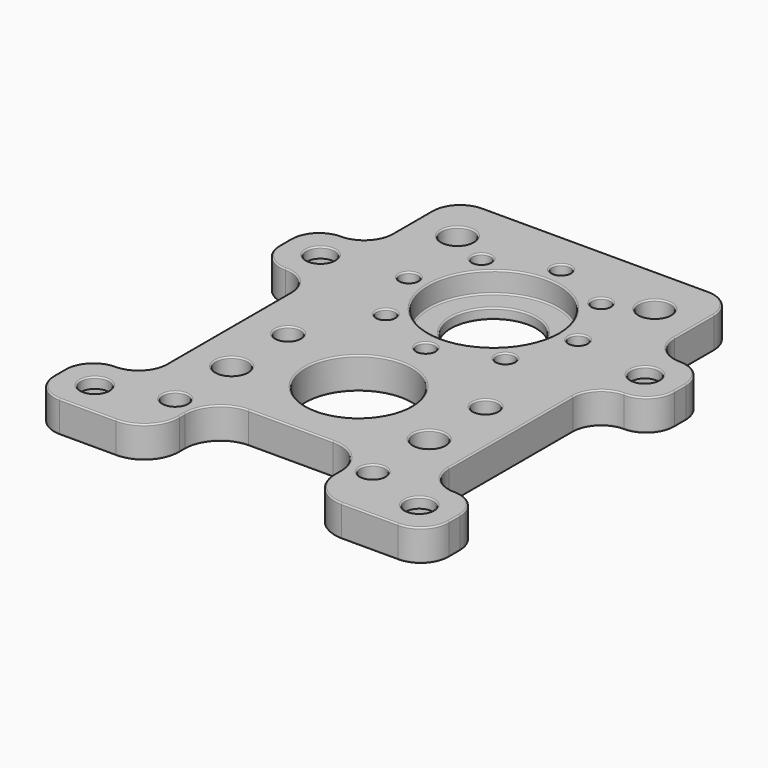
from build123d import *

# Parameters (mm, degrees)
F0_R     = 2.25
F0_R_2   = 1.75
F0_R_3   = 7.5
F0_R_4   = 6
F0_W     = 8
F0_H     = 10
F0_R_5   = 2
F1_DEPTH = 4.5
F2_R     = 1.3
F3_DEPTH = 25
F4_R     = 9.25
F4_R_2   = 6
F5_DEPTH = 3
F6_R     = 3.99999
F7_R     = 3.25
F8_DEPTH = 3
F9_R     = 5
F10_R    = 0.2


# Not quite as in the source:
# - a fillet or chamfer is up to 0.001 mm smaller than in the source, because OpenCascade refuses the exact size
# - a feature names something its author has since deleted; it is built from what else it names


with BuildPart() as f1:
    # F0 (on Top) → F1 (new body)
    with BuildSketch(Plane.XY):
        Polygon((11, -27), (20, -27), (20, 2), (20, 12), (20, 27), (-20, 27), (-20, 12), (-20, 2), (-20, -27), (-11, -27), align=None)
        with Locations((-14, -20)):
            Circle(F0_R, mode=Mode.SUBTRACT)
        with Locations((-14, -10)):
            Circle(F0_R_2, mode=Mode.SUBTRACT)
        with Locations((0, -15)):
            Circle(F0_R_3, mode=Mode.SUBTRACT)
        with Locations((14, -20)):
            Circle(F0_R, mode=Mode.SUBTRACT)
        with Locations((14, -10)):
            Circle(F0_R_2, mode=Mode.SUBTRACT)
        with Locations((-14, 20)):
            Circle(F0_R, mode=Mode.SUBTRACT)
        with Locations((0, 8.9)):
            Circle(F0_R_4, mode=Mode.SUBTRACT)
        with Locations((14, 20)):
            Circle(F0_R, mode=Mode.SUBTRACT)
        Polygon((-11, -30), (-11, -27), (-20, -27), (-20, -28), (-20, -38), (-11, -38), align=None)
        with Locations((-14, -30)):
            Circle(F0_R_2, mode=Mode.SUBTRACT)
        Polygon((20, -28), (20, -27), (11, -27), (11, -30), (11, -38), (20, -38), align=None)
        with Locations((14, -30)):
            Circle(F0_R_2, mode=Mode.SUBTRACT)
        with Locations((-24, 7)):
            Rectangle(F0_W, F0_H)
        with Locations((-23, 7)):
            Circle(F0_R_5, mode=Mode.SUBTRACT)
        with Locations((24, 7)):
            Rectangle(F0_W, F0_H)
        with Locations((23, 7)):
            Circle(F0_R_5, mode=Mode.SUBTRACT)
        with Locations((24, -33)):
            Rectangle(F0_W, F0_H)
        with Locations((23, -33)):
            Circle(F0_R_5, mode=Mode.SUBTRACT)
        with Locations((-24, -33)):
            Rectangle(F0_W, F0_H)
        with Locations((-23, -33)):
            Circle(F0_R_5, mode=Mode.SUBTRACT)
    extrude(amount=F1_DEPTH)

    # F2 (on face) → F3 (cut)
    with BuildSketch(Plane.XY.offset(4.5)):
        with Locations((0, 20.9)):
            Circle(F2_R)
        with Locations((-8.4852813742, 17.3852813742)):
            Circle(F2_R)
        with Locations((-12, 8.9)):
            Circle(F2_R)
        with Locations((-8.4852813742, 0.4147186258)):
            Circle(F2_R)
        with Locations((0, -3.1)):
            Circle(F2_R)
        with Locations((8.4852813742, 0.4147186258)):
            Circle(F2_R)
        with Locations((12, 8.9)):
            Circle(F2_R)
        with Locations((8.4852813742, 17.3852813742)):
            Circle(F2_R)
    extrude(amount=-F3_DEPTH, mode=Mode.SUBTRACT)

    # F4 (on face) → F5 (cut)
    with BuildSketch(Plane.XY.offset(4.5)):
        with Locations((0, 8.9)):
            Circle(F4_R)
        with Locations((0, 8.9)):
            Circle(F4_R_2, mode=Mode.SUBTRACT)
    extrude(amount=-F5_DEPTH, mode=Mode.SUBTRACT)

    # F6 (radius 4 in the source; OpenCascade refuses exactly that, so slightly less here)
    f6_edges = [f1.edges().sort_by_distance(p)[0] for p in [
        (-28, -38, 2.25),
        (28, 12, 2.25),
        (28, -28, 2.25),
        (28, -38, 2.25),
        (-20, 2, 2.25),
        (-20, -28, 2.25),
        (28, 2, 2.25),
        (-20, 27, 2.25),
        (-20, 12, 2.25),
        (20, -28, 2.25),
        (-28, -28, 2.25),
        (20, 2, 2.25),
        (-28, 2, 2.25),
        (20, 12, 2.25),
        (-28, 12, 2.25),
        (20, 27, 2.25),
    ]]
    fillet(f6_edges, radius=F6_R)

    # F7 (on face) → F8 (cut)
    with BuildSketch(Plane(origin=(0, 0, 0), x_dir=(1, 0, 0), z_dir=(0, 0, -1))):
        with Locations((23, -7)):
            Circle(F7_R)
        with Locations((23, 33)):
            Circle(F7_R)
        with Locations((-23, -7)):
            Circle(F7_R)
        with Locations((-23, 33)):
            Circle(F7_R)
    extrude(amount=-F8_DEPTH, mode=Mode.SUBTRACT)

    # F9
    f9_edges = [f1.edges().sort_by_distance(p)[0] for p in [
        (-11, -27, 2.25),
        (-11, -38, 2.25),
        (11, -27, 2.25),
        (11, -38, 2.25),
    ]]
    fillet(f9_edges, radius=F9_R)

    # F10
    f10_edges = [f1.edges().sort_by_distance(p)[0] for p in [
        (20.000005, -38, 0),
        (12.464466, -36.535534, 0),
        (26.82843, -36.82843, 0),
        (11, -32.5, 0),
        (28, -33, 0),
        (9.535534, -28.464466, 0),
        (26.82843, -29.17157, 0),
        (0, -27, 0),
        (24, -28, 0),
        (-9.535534, -28.464466, 0),
        (21.17157, -26.82843, 0),
        (-11, -32.5, 0),
        (20, -13, 0),
        (-12.464466, -36.535534, 0),
        (21.17157, 0.82843, 0),
        (-20.000005, -38, 0),
        (24, 2, 0),
        (-26.82843, -36.82843, 0),
        (26.82843, 3.17157, 0),
        (-28, -33, 0),
        (28, 7, 0),
        (-26.82843, -29.17157, 0),
        (26.82843, 10.82843, 0),
        (-24, -28, 0),
        (24, 12, 0),
        (-21.17157, -26.82843, 0),
        (21.17157, 13.17157, 0),
        (-20, -13, 0),
        (20, 19.5, 0),
        (-21.17157, 0.82843, 0),
        (18.82843, 25.82843, 0),
        (-24, 2, 0),
        (0, 27, 0),
        (-26.82843, 3.17157, 0),
        (-18.82843, 25.82843, 0),
        (-28, 7, 0),
        (-20, 19.5, 0),
        (-26.82843, 10.82843, 0),
        (-21.17157, 13.17157, 0),
        (-24, 12, 0),
        (-26.25, -33, 0),
        (-15.75, -30, 0),
        (-16.25, -20, 0),
        (-15.75, -10, 0),
        (12.25, -30, 0),
        (19.75, -33, 0),
        (-7.5, -15, 0),
        (11.75, -20, 0),
        (12.25, -10, 0),
        (-26.25, 7, 0),
        (-9.785281, 0.414719, 0),
        (-16.25, 20, 0),
        (-13.3, 8.9, 0),
        (-9.785281, 17.385281, 0),
        (-1.3, -3.1, 0),
        (7.185281, 0.414719, 0),
        (19.75, 7, 0),
        (-6, 8.9, 0),
        (10.7, 8.9, 0),
        (-1.3, 20.9, 0),
        (7.185281, 17.385281, 0),
        (11.75, 20, 0),
        (20.000005, -38, 4.5),
        (12.464466, -36.535534, 4.5),
        (26.82843, -36.82843, 4.5),
        (11, -32.5, 4.5),
        (28, -33, 4.5),
        (9.535534, -28.464466, 4.5),
        (26.82843, -29.17157, 4.5),
        (0, -27, 4.5),
        (24, -28, 4.5),
        (-9.535534, -28.464466, 4.5),
        (21.17157, -26.82843, 4.5),
        (-11, -32.5, 4.5),
        (20, -13, 4.5),
        (-12.464466, -36.535534, 4.5),
        (21.17157, 0.82843, 4.5),
        (-20.000005, -38, 4.5),
        (24, 2, 4.5),
        (-26.82843, -36.82843, 4.5),
        (26.82843, 3.17157, 4.5),
        (-28, -33, 4.5),
        (28, 7, 4.5),
        (-26.82843, -29.17157, 4.5),
        (26.82843, 10.82843, 4.5),
        (-24, -28, 4.5),
        (24, 12, 4.5),
        (-21.17157, -26.82843, 4.5),
        (21.17157, 13.17157, 4.5),
        (-20, -13, 4.5),
        (20, 19.5, 4.5),
        (-21.17157, 0.82843, 4.5),
        (18.82843, 25.82843, 4.5),
        (-24, 2, 4.5),
        (0, 27, 4.5),
        (-26.82843, 3.17157, 4.5),
        (-18.82843, 25.82843, 4.5),
        (-28, 7, 4.5),
        (-20, 19.5, 4.5),
        (-26.82843, 10.82843, 4.5),
        (-21.17157, 13.17157, 4.5),
        (-24, 12, 4.5),
        (-25, -33, 4.5),
        (-15.75, -30, 4.5),
        (-16.25, -20, 4.5),
        (-15.75, -10, 4.5),
        (12.25, -30, 4.5),
        (21, -33, 4.5),
        (-7.5, -15, 4.5),
        (11.75, -20, 4.5),
        (12.25, -10, 4.5),
        (-25, 7, 4.5),
        (-9.785281, 0.414719, 4.5),
        (-16.25, 20, 4.5),
        (-13.3, 8.9, 4.5),
        (-9.785281, 17.385281, 4.5),
        (-1.3, -3.1, 4.5),
        (7.185281, 0.414719, 4.5),
        (21, 7, 4.5),
        (-9.25, 8.9, 4.5),
        (10.7, 8.9, 4.5),
        (-1.3, 20.9, 4.5),
        (7.185281, 17.385281, 4.5),
        (11.75, 20, 4.5),
        (-9.25, 8.9, 1.5),
        (-6, 8.9, 1.5),
    ]]
    fillet(f10_edges, radius=F10_R)


solid = f1.part
